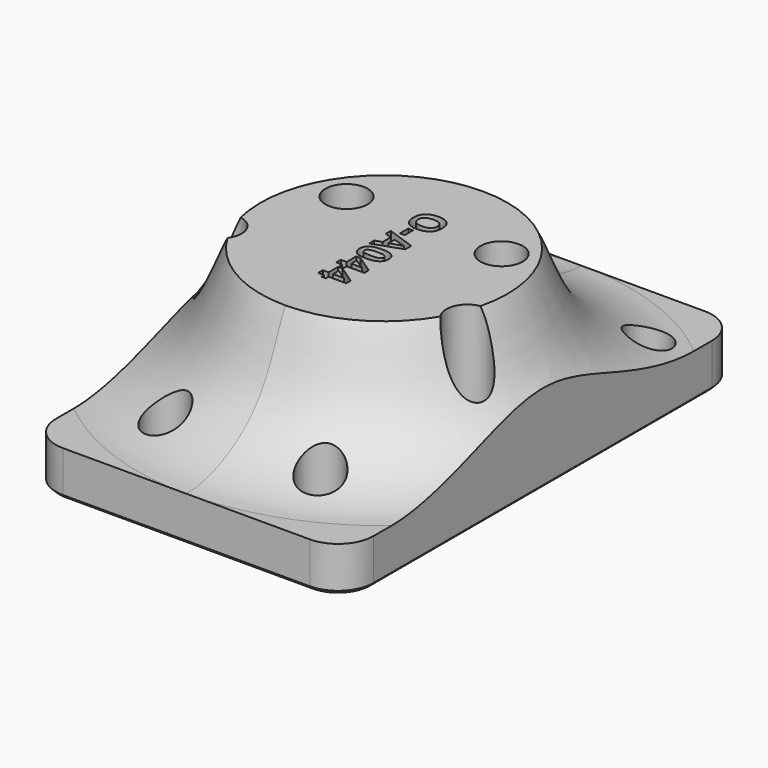
from build123d import *

# Parameters (mm, degrees)
F0_W         = 22.5
F0_H         = 70
F0_R         = 3
F1_DEPTH     = 22.75
F2_R         = 5
F3_SIZE      = 0.5
F4_W         = 20.8567456901
F4_H         = 16.4
F7_TEXT_SIZE = 5.6034671453
F8_DEPTH     = 1.5


# Not quite as in the source:
# - Text() gives the source's letters only with a copy of the font that has no kerning and outlines rounded to 1/6400 em; it was checked with that copy


with BuildPart() as f1:
    # F0 (on Top) → F1 (new body)
    with BuildSketch(Plane.XY):
        with Locations((-11.25, 0)):
            Rectangle(F0_W, F0_H)
        with Locations((-10.9845162696, -25)):
            Circle(F0_R, mode=Mode.SUBTRACT)
        with Locations((-17.5, -7.098855574)):
            Circle(F0_R, mode=Mode.SUBTRACT)
        with Locations((-10.9845162696, 7.098855574)):
            Circle(F0_R, mode=Mode.SUBTRACT)
        with Locations((-17.5, 25)):
            Circle(F0_R, mode=Mode.SUBTRACT)
    extrude(amount=F1_DEPTH)

    # F2
    f2_edges = [f1.edges().sort_by_distance(p)[0] for p in [
        (-22.5, -35, 11.375),
        (-22.5, 35, 11.375),
    ]]
    fillet(f2_edges, radius=F2_R)

    # F3
    f3_edges = [f1.edges().sort_by_distance(p)[0] for p in [
        (-8.75, 35, 0),
        (-22.5, 0, 0),
        (-8.75, -35, 0),
    ]]
    chamfer(f3_edges, length=F3_SIZE)

    # F4 (on face) → F5 (revolve, cut)
    with BuildSketch(Plane.YZ):
        with Locations((-45.4283728451, 14.55)):
            Rectangle(F4_W, F4_H)
        with BuildLine():
            add(Edge.make_bspline(
                [(-35, 6.35), (-30.8567456901, 6.35), (-21.3478268247, 10.6342936928), (-19, 19.75), (-17.5, 22.75)],
                knots=[0, 0, 0, 0, 0.5117304725, 1, 1, 1, 1], degree=3))
            Line((-17.5, 22.75), (-35, 22.75))
            Line((-35, 22.75), (-35, 6.35))
        make_face()
    revolve(axis=Axis((0, 0, 2.9836259782), (0, 0, -1)), mode=Mode.SUBTRACT)

    # F6: F1 across plane


with BuildPart() as f1_1:
    add(f1.part)
    add(f1.part.mirror(Plane.YZ))

    # F7 (on face) → F8 (cut)
    with BuildSketch(Plane.XY.offset(22.75)):
        with Locations(Location((-2.0172481723, 10), (0, 0, -90))):
            Text('O-A044', F7_TEXT_SIZE, font='Open Sans', font_style=FontStyle.BOLD, text_align=(TextAlign.LEFT, TextAlign.BOTTOM))
    extrude(amount=-F8_DEPTH, mode=Mode.SUBTRACT)


solid = f1_1.part
